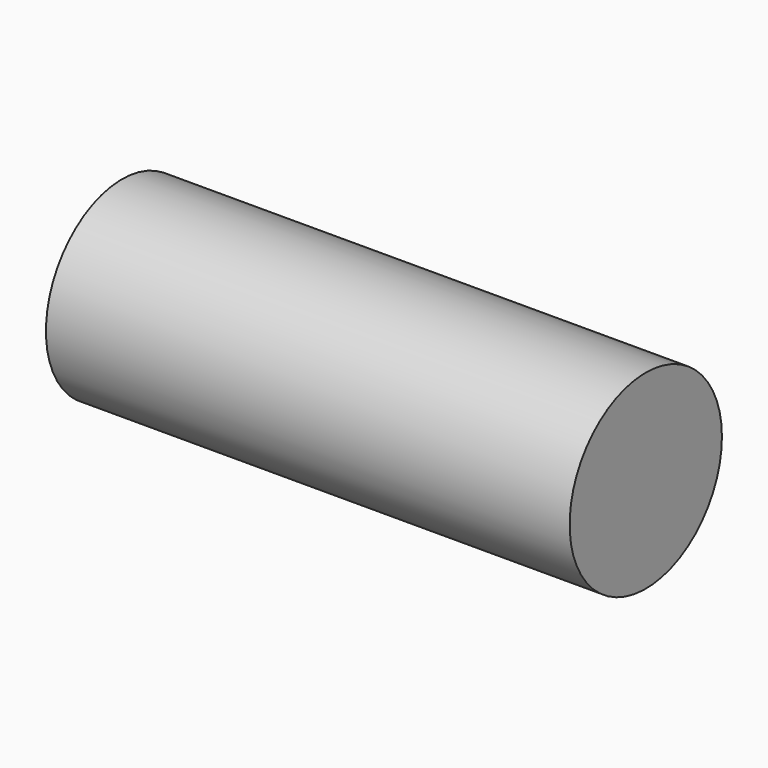
from build123d import *

# Parameters (mm, degrees)
F2_R     = 28.662672352
F3_DEPTH = 157.734


# Not quite as in the source:
# - the program builds the solid bodies; features that only make, move or delete a surface that nothing else refers to are left out


with BuildPart() as f3:
    # F2 (on Right) → F3 (new body)
    with BuildSketch(Plane.YZ):
        with Locations((53.9907179773, 0)):
            Circle(F2_R)
    extrude(amount=-F3_DEPTH)


solid = f3.part
